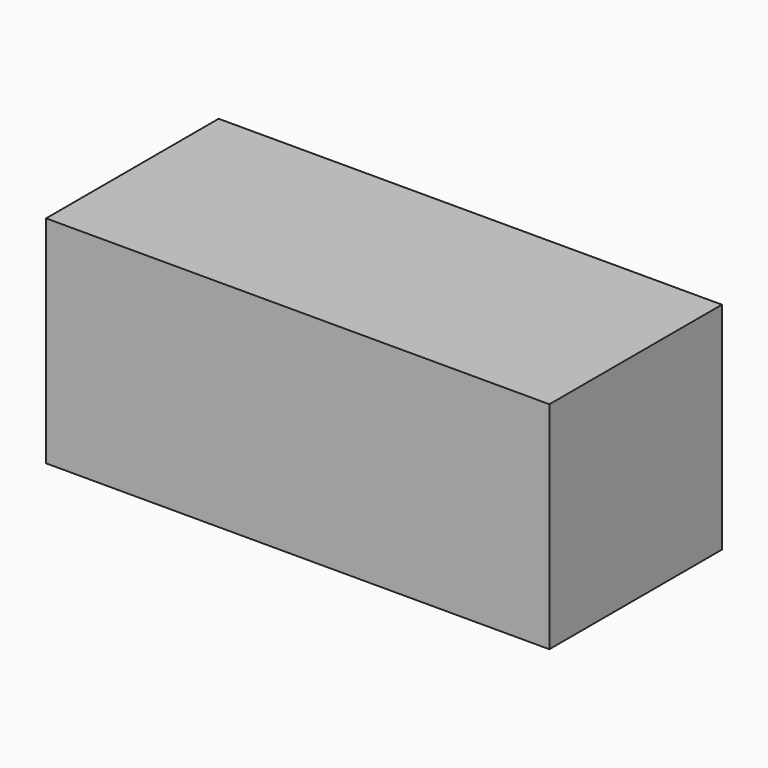
from build123d import *

# Parameters (mm, degrees)
F0_W     = 140
F0_H     = 60
F1_DEPTH = 60


# Not quite as in the source:
# - the program builds the solid bodies; features that only make, move or delete a surface that nothing else refers to are left out


with BuildPart() as f1:
    # F0 (on Top) → F1 (new body)
    with BuildSketch(Plane.XY):
        Rectangle(F0_W, F0_H)
    extrude(amount=F1_DEPTH)


solid = f1.part
